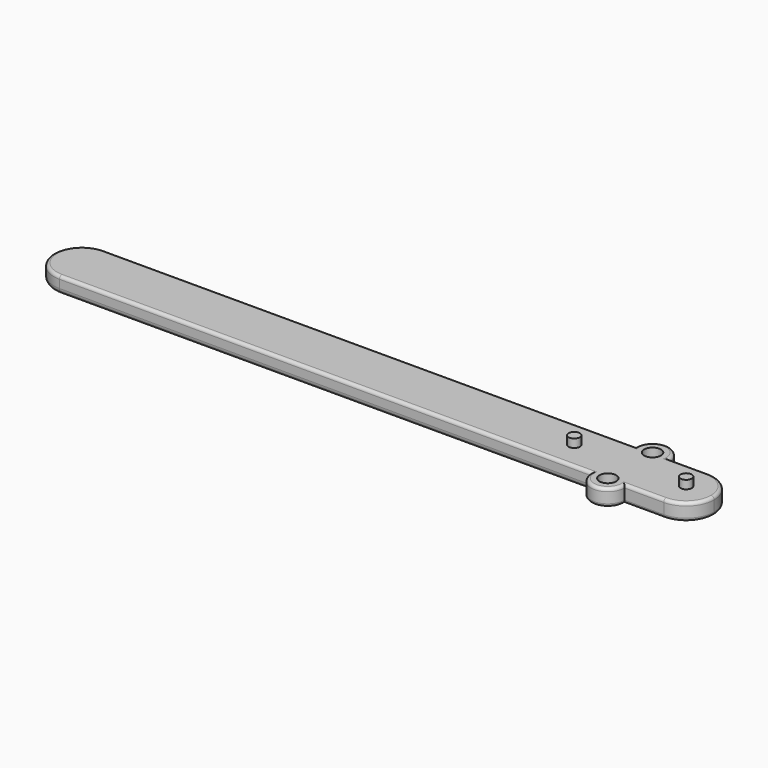
from build123d import *
from build123d import SkipClean  # not in build123d's __all__

# Parameters (mm, degrees)
F0_R     = 1.5
F1_DEPTH = 3
F2_R     = 0.55
F3_R     = 1
F4_R     = 0.5499
F5_R     = 1
F6_DEPTH = 4.5


# Not quite as in the source:
# - a fillet or chamfer is up to 0.001 mm smaller than in the source, because OpenCascade refuses the exact size
# - a feature names something its author has since deleted; it is built from what else it names


with BuildPart() as f1:
    # F0 (on Top) → F1 (new body)
    with BuildSketch(Plane.XY):
        with BuildLine():
            Line((-95, 0), (0, 0))
            ThreePointArc((0, 0), (3, -3), (6, 0))
            Line((6, 0), (13, 0))
            ThreePointArc((13, 0), (16.5355339059, 1.4644660941), (18, 5))
            ThreePointArc((18, 5), (16.5355339059, 8.5355339059), (13, 10))
            Line((13, 10), (6, 10))
            ThreePointArc((6, 10), (3, 13), (0, 10))
            Line((0, 10), (-95, 10))
            ThreePointArc((-95, 10), (-98.5355339059, 8.5355339059), (-100, 5))
            ThreePointArc((-100, 5), (-98.5355339059, 1.4644660941), (-95, 0))
        make_face()
        with Locations((3, 0)):
            Circle(F0_R, mode=Mode.SUBTRACT)
        with Locations((3, 10)):
            Circle(F0_R, mode=Mode.SUBTRACT)
    extrude(amount=F1_DEPTH)

    # F2
    f2_edges = [f1.edges().sort_by_distance(p)[0] for p in [
        (-47.5, 0, 3),
    ]]
    fillet(f2_edges, radius=F2_R)

    # F3
    f3_edges = [f1.edges().sort_by_distance(p)[0] for p in [
        (-47.5, 0, 0),
    ]]
    fillet(f3_edges, radius=F3_R)

    # F4 (radius 0.55 in the source; OpenCascade refuses exactly that, so slightly less here)
    f4_edges = [f1.edges().sort_by_distance(p)[0] for p in [
        (3, -3, 3),
        (3, 13, 3),
        (3, -3, 0),
        (3, 13, 0),
        (9.5, 0, 3),
        (18, 5, 3),
        (18, 5, 0),
        (9.5, 0, 0),
        (9.5, 10, 0),
        (9.5, 10, 3),
    ]]
    fillet(f4_edges, radius=F4_R)

    # F5 (on Top) → F6 (join)
    with BuildSketch(Plane.XY):
        with Locations((12.9994759336, 5.0007845275)):
            Circle(F5_R)
        with Locations((-6.9997087121, 5.0000692718)):
            Circle(F5_R)
    with SkipClean():  # cleaning this boolean's faces spoils the solid; the shape is the same uncleaned
        extrude(amount=F6_DEPTH)


solid = f1.part
